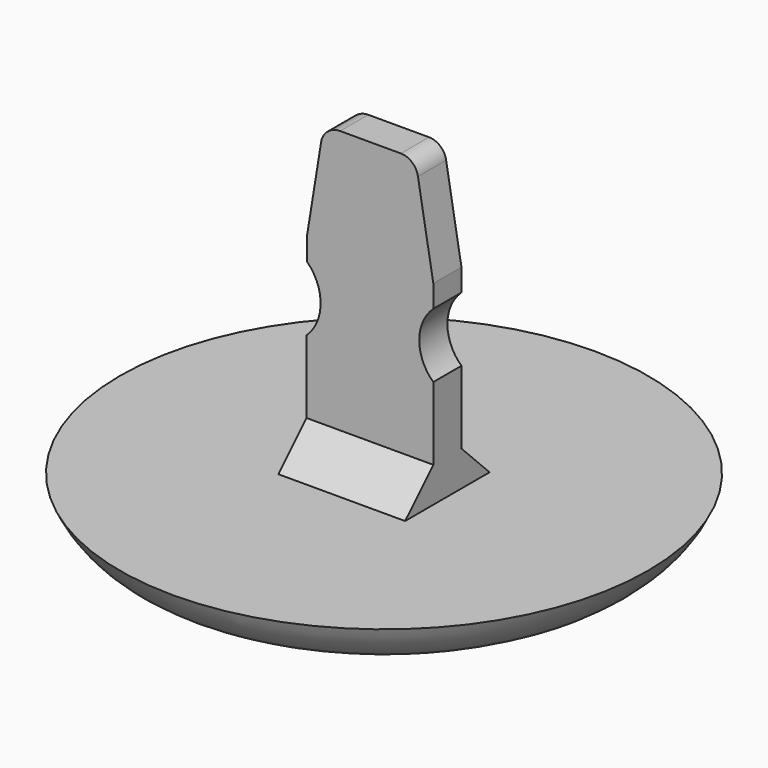
from build123d import *

# Parameters (mm, degrees)
F1_DEPTH = 2
F2_R     = 15
F2_W     = 7.199677173
F2_H     = 2
F3_DEPTH = 3
F4_W     = 7.199677173
F4_H     = 2
F5_DEPTH = 2
F6_SIZE  = 1.99999
F7_W     = 7.199677173
F7_H     = 2
F8_DEPTH = 2
F9_SIZE  = 1.99999


# Not quite as in the source:
# - a fillet or chamfer that OpenCascade refuses, or shapes differently, is made with other operations: its cross-section is extruded or revolved along the edge and cut away or added
# - a fillet or chamfer is up to 0.001 mm smaller than in the source, because OpenCascade refuses the exact size


with BuildPart() as f1:
    # F0 (on Front) → F1 (new body)
    with BuildSketch(Plane.XZ):
        with BuildLine():
            ThreePointArc((-1.6914953012, 28.8060177118), (-2.3588223185, 28.5823009391), (-2.7564610355, 28.0015617609))
            Line((-2.7564610355, 28.0015617609), (-3.5831569694, 22.9014810175))
            Line((-3.5831569694, 22.9014810175), (-3.5831569694, 21.6677952558))
            ThreePointArc((-3.5831569694, 21.6677952558), (-2.8004223212, 19.8132576007), (-3.6002863199, 17.9660432041))
            Line((-3.6002863199, 17.9660432041), (-3.6002863199, 11.8300495669))
            Line((-3.6002863199, 11.8300495669), (3.5993908532, 11.8300495669))
            Line((3.5993908532, 11.8300495669), (3.5993908532, 17.969943583))
            ThreePointArc((3.5993908532, 17.969943583), (2.8023887863, 19.8030117696), (3.6017470993, 21.6350536793))
            Line((3.6017470993, 21.6350536793), (3.6017470993, 22.9016747326))
            Line((3.6017470993, 22.9016747326), (2.7295136824, 27.9675517231))
            ThreePointArc((2.7295136824, 27.9675517231), (2.3994359185, 28.5674317792), (1.7576538958, 28.8060177118))
            Line((1.7576538958, 28.8060177118), (-1.6914953012, 28.8060177118))
        make_face()
    extrude(amount=F1_DEPTH)

    # F2 (on face) → F3 (join)
    with BuildSketch(Plane(origin=(0, 0, 11.8300495669), x_dir=(1, 0, 0), z_dir=(0, 0, -1))):
        with Locations((0, 1)):
            Circle(F2_R)
        with Locations((-0.0004477333, 1)):
            Rectangle(F2_W, F2_H, mode=Mode.SUBTRACT)
        with Locations((-0.0004477333, 1)):
            Rectangle(F2_W, F2_H)
    extrude(amount=F3_DEPTH)

    # F4 (on face) → F5 (join)
    with BuildSketch(Plane(origin=(0, 0, 0), x_dir=(-1, 0, 0), z_dir=(0, 1, 0))):
        with Locations((0.0004477333, 12.8300495669)):
            Rectangle(F4_W, F4_H)
    extrude(amount=F5_DEPTH)

    # F6 (size 2 in the source; OpenCascade refuses exactly that, so slightly less here)
    f6_edges = [f1.edges().sort_by_distance(p)[0] for p in [
        (-0.000448, 2, 13.83005),
    ]]
    chamfer(f6_edges, length=F6_SIZE)

    # F7 (on face) → F8 (join)
    with BuildSketch(Plane.XZ.offset(2)):
        with Locations((-0.0004477333, 12.8300495669)):
            Rectangle(F7_W, F7_H)
    extrude(amount=F8_DEPTH)

    # F9 (size 2 in the source; OpenCascade refuses exactly that, so slightly less here)
    f9_edges = [f1.edges().sort_by_distance(p)[0] for p in [
        (-0.000448, -4, 13.83005),
    ]]
    chamfer(f9_edges, length=F9_SIZE)

    # F10: fillet of radius 5 on 1 edges, made by hand

    # F10_s1 → F10_t2 (revolve, cut)
    with BuildSketch(Plane.XZ.offset(1)):
        with BuildLine():
            ThreePointArc((15, 11.8300495669), (13.1560370926, 9.6467494343), (10.417424305, 8.8300495669))
            Line((10.417424305, 8.8300495669), (15, 8.8300495669))
            Line((15, 8.8300495669), (15, 11.8300495669))
        make_face()
    revolve(axis=Axis((0, -1, 8.8300495669), (0, 0, -1)), mode=Mode.SUBTRACT)


solid = f1.part
